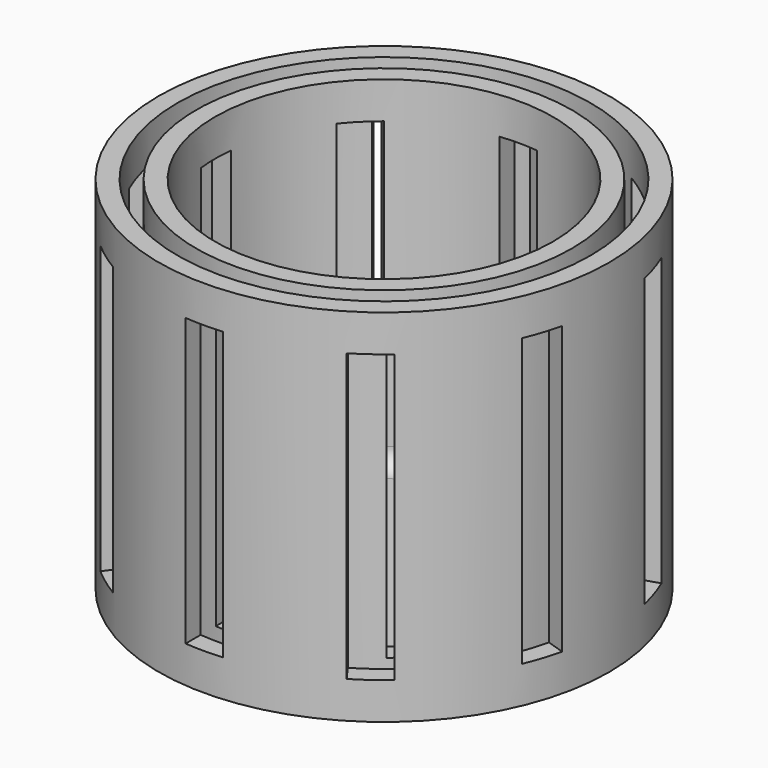
from build123d import *

# Parameters (mm, degrees)
F2_W            = 10
F2_H            = 76.3443418741
F3_REACH        = 136.997483921
F3_COPIES_COUNT = 8
F5_W            = 10
F5_H            = 76.3443418741
F6_REACH        = 211.997483921
F6_COPIES_COUNT = 10


# Not quite as in the source:
# - a pattern or mirror of a feature is missing from the dataset's text; its kind, count and spacing are read off the source's solid


with BuildPart() as f1:
    # F0 (on Front) → F1 (revolve)
    with BuildSketch(Plane.XZ):
        with BuildLine():
            Line((0, 5), (0, 0))
            Line((0, 0), (60, 0))
            Line((60, 0), (60, 96))
            Line((60, 96), (55, 96))
            Line((55, 96), (55, 5))
            Line((55, 5), (50, 5))
            Line((50, 5), (50, 96))
            Line((50, 96), (45, 96))
            Line((45, 96), (45, 10))
            ThreePointArc((45, 10), (43.5355339059, 6.4644660941), (40, 5))
            Line((40, 5), (0, 5))
        make_face()
    revolve(axis=Axis((0, 0, 2.5), (0, 0, 1)))

    f3_end = f1.faces().sort_by_distance((-50, 0, 50.5))[0]
    # F2 (on Front) → F3 (cut, up to a face of the model that its end follows)
    with BuildSketch(Plane.XZ):
        with Locations((0, 48)):
            Rectangle(F2_W, F2_H)
    f3_long = extrude(amount=F3_REACH, mode=Mode.PRIVATE)
    f3 = split(f3_long, bisect_by=f3_end, keep=Keep.BOTTOM, mode=Mode.PRIVATE)
    add(f3, mode=Mode.SUBTRACT)

    # F3_copies: F3 ×8 about axis
    f3_copies_axis = Axis((0, 0, 0), (0, 0, 1))
    for i in range(1, F3_COPIES_COUNT):
        add(f3.rotate(f3_copies_axis, i * 360 / F3_COPIES_COUNT), mode=Mode.SUBTRACT)

    f6_end = f1.faces().sort_by_distance((-55, 0, 50.5))[0]
    # F5 (on offset) → F6 (cut, up to a face of the model that its end follows)
    with BuildSketch(Plane.XZ.offset(75)):
        with Locations((0, 48)):
            Rectangle(F5_W, F5_H)
    f6_long = extrude(amount=-F6_REACH, mode=Mode.PRIVATE)
    f6 = split(f6_long, bisect_by=f6_end, keep=Keep.ALL, mode=Mode.PRIVATE).solids().sort_by_distance((0, -75, 48))[0]
    add(f6, mode=Mode.SUBTRACT)

    # F6_copies: F6 ×10 about axis
    f6_copies_axis = Axis((0, 0, 0), (0, 0, 1))
    for i in range(1, F6_COPIES_COUNT):
        add(f6.rotate(f6_copies_axis, i * 360 / F6_COPIES_COUNT), mode=Mode.SUBTRACT)


solid = f1.part
